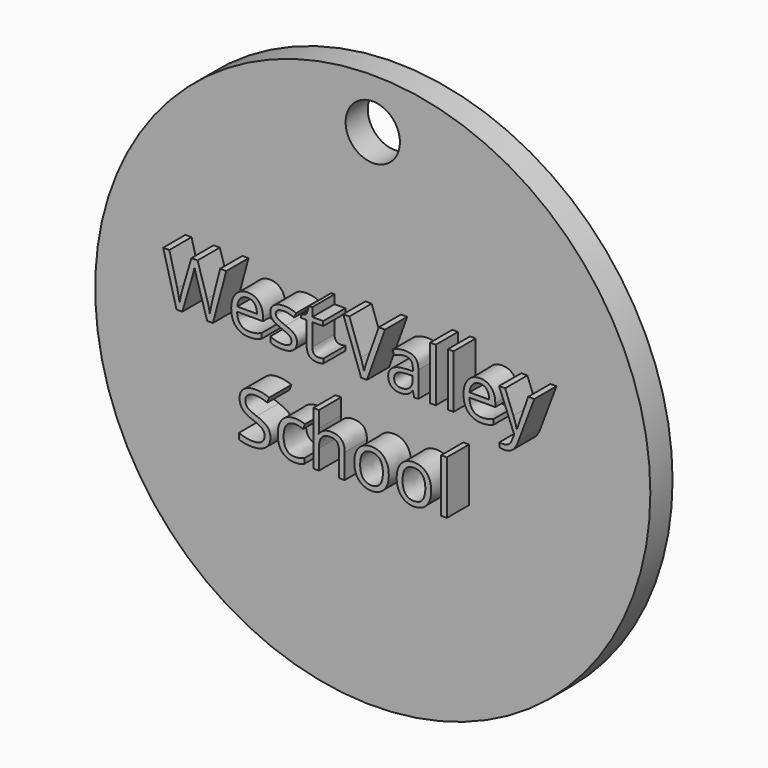
from build123d import *

# Parameters (mm, degrees)
F0_R         = 31.75
F1_DEPTH     = 3.175
F2_TEXT_SIZE = 8.0310534792
F3_DEPTH     = 3.175
F4_R         = 3.1054418037
F5_DEPTH     = 12.7


# Not quite as in the source:
# - Text() gives the source's letters only with a copy of the font that has no kerning and outlines rounded to 1/6400 em; it was checked with that copy


with BuildPart() as f1:
    # F0 (on Front) → F1 (new body)
    with BuildSketch(Plane.XZ):
        Circle(F0_R)
    extrude(amount=F1_DEPTH)

    # F2 (on face) → F3 (join)
    with BuildSketch(Plane.XZ.offset(3.175)):
        with Locations((-21.5345169931, 2.9542625416)):
            Text('West Valley', F2_TEXT_SIZE, font='Open Sans', text_align=(TextAlign.LEFT, TextAlign.BOTTOM))
        with Locations((-13.1872407832, -7.96797019)):
            Text('School', F2_TEXT_SIZE, font='Open Sans', text_align=(TextAlign.LEFT, TextAlign.BOTTOM))
    extrude(amount=F3_DEPTH)

    # F4 (on face) → F5 (cut, symmetric)
    with BuildSketch(Plane.XZ.offset(3.175)):
        with Locations((0, 26.0002948344)):
            Circle(F4_R)
    extrude(amount=F5_DEPTH, both=True, mode=Mode.SUBTRACT)


solid = f1.part
